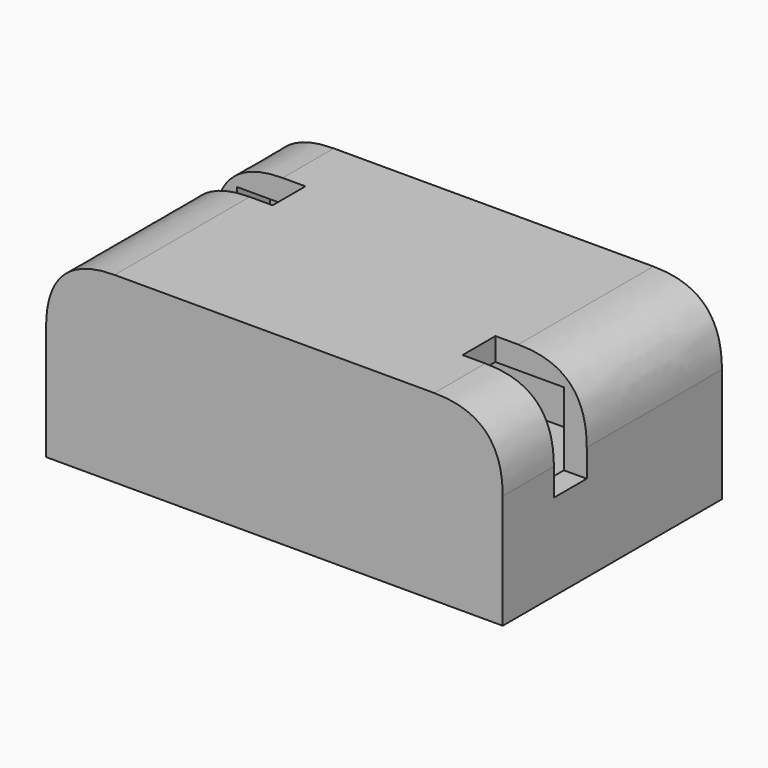
from build123d import *

# Parameters (mm, degrees)
F0_W        = 254
F0_H        = 177.8
F1_DEPTH    = 152.4
F2_T        = -12.7
F3_T1_DEPTH = 342.9
F4_T1_DEPTH = 342.9
F5_W        = 22.86
F5_H        = 83.3190586418
F6_DEPTH    = 50.8
F7_W        = 22.86
F7_H        = 76.2
F8_DEPTH    = 50.8
F9_W        = 50.8
F9_H        = 25.4
F10_DEPTH   = 233.68
F11_W       = 254
F11_H       = 76.2
F12_DEPTH   = 180.34


# Not quite as in the source:
# - a fillet or chamfer that OpenCascade refuses, or shapes differently, is made with other operations: its cross-section is extruded or revolved along the edge and cut away or added


with BuildPart() as f1:
    # F0 (on Front) → F1 (new body)
    with BuildSketch(Plane.XZ):
        with Locations((61.0858832002, 0.9791328073)):
            Rectangle(F0_W, F0_H)
    extrude(amount=F1_DEPTH)

    # F2
    f2_openings = [f1.faces().sort_by_distance(p)[0] for p in [
        (61.085883, -76.2, -87.920867),
    ]]
    offset(amount=F2_T, openings=f2_openings)

    # F3: fillet of radius 38.1 on 1 edges, made by hand

    # F3_s2 → F3_t1 (cut)
    with BuildSketch(Plane.XZ.offset(-95.25)):
        with BuildLine():
            add(Edge.make_bspline(
                [(188.0858832002, 51.7791328073), (188.0858832002, 89.8791328073), (149.9858832002, 89.8791328073)],
                knots=[0, 0, 0, 1, 1, 1], degree=2, weights=[1, 1, 1]))
            Line((149.9858832002, 89.8791328073), (188.0858832002, 89.8791328073))
            Line((188.0858832002, 89.8791328073), (188.0858832002, 51.7791328073))
        make_face()
    extrude(amount=F3_T1_DEPTH, mode=Mode.SUBTRACT)

    # F4: fillet of radius 38.1 on 1 edges, made by hand

    # F4_s2 → F4_t1 (cut)
    with BuildSketch(Plane.XZ.offset(-95.25)):
        with BuildLine():
            add(Edge.make_bspline(
                [(-65.9141167998, 51.7791328073), (-65.9141167998, 89.8791328073), (-27.8141167998, 89.8791328073)],
                knots=[0, 0, 0, 1, 1, 1], degree=2, weights=[1, 1, 1]))
            Line((-27.8141167998, 89.8791328073), (-65.9141167998, 89.8791328073))
            Line((-65.9141167998, 89.8791328073), (-65.9141167998, 51.7791328073))
        make_face()
    extrude(amount=F4_T1_DEPTH, mode=Mode.SUBTRACT)

    # F5 (on face) → F6 (cut)
    with BuildSketch(Plane(origin=(-65.9141167998, 0, 0), x_dir=(0, -1, 0), z_dir=(-1, 0, 0))):
        with Locations((46.99, 78.1986621282)):
            Rectangle(F5_W, F5_H)
    extrude(amount=-F6_DEPTH, mode=Mode.SUBTRACT)

    # F7 (on face) → F8 (cut)
    with BuildSketch(Plane.YZ.offset(188.0858832002)):
        with Locations((-105.41, 74.6391328073)):
            Rectangle(F7_W, F7_H)
    extrude(amount=-F8_DEPTH, mode=Mode.SUBTRACT)

    # F9 (on face) → F10 (join)
    with BuildSketch(Plane(origin=(175.3858832002, 0, 0), x_dir=(0, -1, 0), z_dir=(-1, 0, 0))):
        with Locations((76.2, 16.2191328073)):
            Rectangle(F9_W, F9_H)
    extrude(amount=F10_DEPTH)

    # F11 (on face) → F12 (cut)
    with BuildSketch(Plane.XZ.offset(152.4)):
        with Locations((61.0858832002, -49.8208671927)):
            Rectangle(F11_W, F11_H)
    extrude(amount=-F12_DEPTH, mode=Mode.SUBTRACT)


solid = f1.part
